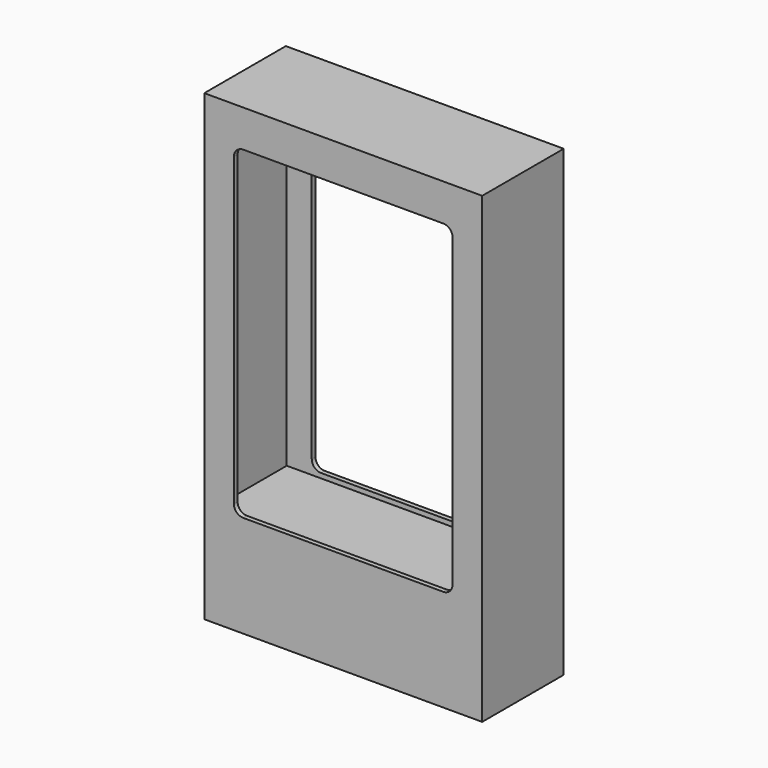
from build123d import *

# Parameters (mm, degrees)
F0_W     = 150
F0_H     = 250
F1_DEPTH = 55
F2_W     = 118
F2_H     = 175
F3_DEPTH = 55.001
F4_R     = 5
F5_T     = -2.5
F6_W     = 145
F6_H     = 49.9277314544
F7_DEPTH = 50


with BuildPart() as f1:
    # F0 (on Front) → F1 (new body)
    with BuildSketch(Plane.XZ):
        with Locations((75, 125)):
            Rectangle(F0_W, F0_H)
    extrude(amount=F1_DEPTH)

    # F2 (on face) → F3 (cut, through all)
    with BuildSketch(Plane.XZ.offset(55)):
        with Locations((75, 142.5)):
            Rectangle(F2_W, F2_H)
    extrude(amount=-F3_DEPTH, mode=Mode.SUBTRACT)

    # F4
    f4_edges = [f1.edges().sort_by_distance(p)[0] for p in [
        (16, -27.5, 230),
        (134, -27.5, 230),
        (134, -27.5, 55),
        (16, -27.5, 55),
    ]]
    fillet(f4_edges, radius=F4_R)

    # F5
    f5_openings = [f1.faces().sort_by_distance(p)[0] for p in [
        (16, -27.5, 142.5),
        (17.464466, -27.5, 56.464466),
        (75, -27.5, 55),
        (132.535534, -27.5, 56.464466),
        (134, -27.5, 142.5),
        (17.464466, -27.5, 228.535534),
        (75, -27.5, 230),
        (132.535534, -27.5, 228.535534),
    ]]
    offset(amount=F5_T, openings=f5_openings)

    # F6 (on face) → F7 (join, through all)
    with BuildSketch(Plane.XZ.offset(2.5)):
        with Locations((75, 27.4638657272)):
            Rectangle(F6_W, F6_H)
    extrude(amount=F7_DEPTH)


solid = f1.part
